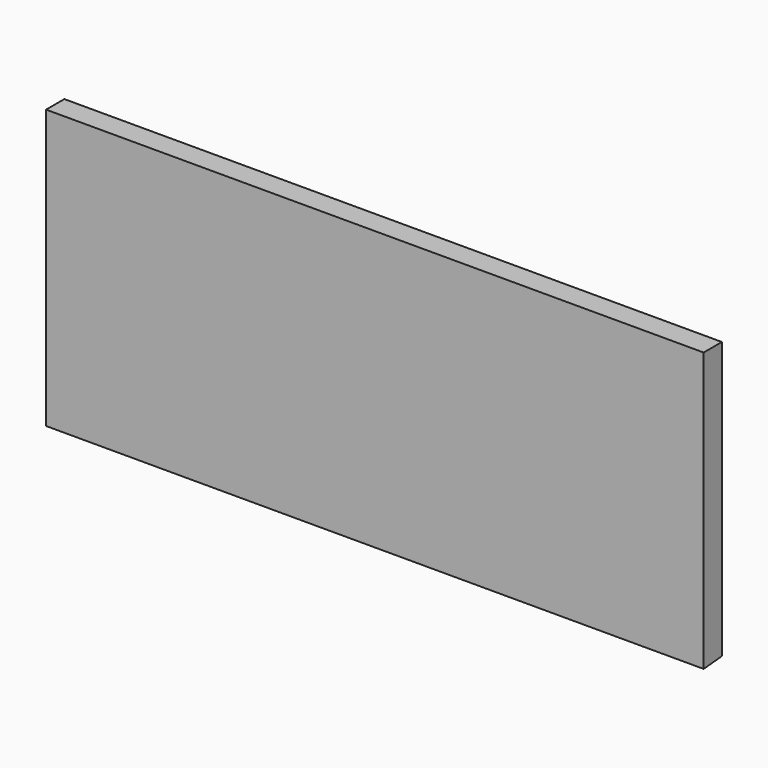
from build123d import *

# Parameters (mm, degrees)
F0_W     = 457.2
F0_H     = 193.675
F1_DEPTH = 15.875
F3_DEPTH = 457.201


# Not quite as in the source:
# - a feature names something its author has since deleted; it is built from what else it names


with BuildPart() as f1:
    # F0 (on Front) → F1 (new body)
    with BuildSketch(Plane.XZ):
        Rectangle(F0_W, F0_H)
    extrude(amount=F1_DEPTH)

    # F2 (on face) → F3 (cut, through all)
    with BuildSketch(Plane.YZ.offset(228.6)):
        Polygon((0, -95.4486174665), (-15.875, -96.8375), (0, -96.8375), align=None)
    extrude(amount=-F3_DEPTH, mode=Mode.SUBTRACT)


solid = f1.part
